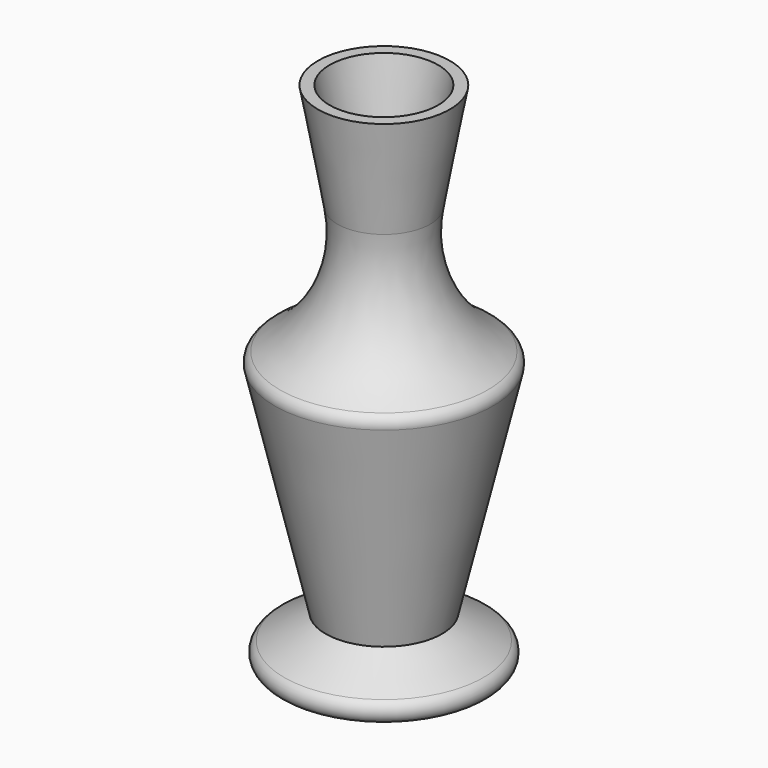
from build123d import *

# Parameters (mm, degrees)
F2_T = -2.54


with BuildPart() as f1:
    # F0 (on Front) → F1 (revolve)
    with BuildSketch(Plane.XZ):
        with BuildLine():
            Line((0, -60.174100101), (0, 52.9934205115))
            Line((0, 52.9934205115), (-14.648579061, 52.9934205115))
            Line((-14.648579061, 52.9934205115), (-10.3401709348, 29.1535649449))
            ThreePointArc((-10.3401709348, 29.1535649449), (-12.3279746399, 13.038394143), (-23.1049332883, 0.8931376273))
            ThreePointArc((-23.1049332883, 0.8931376273), (-24.1326249422, -0.2958024436), (-24.264081516, -1.8618317527))
            Line((-24.264081516, -1.8618317527), (-12.9252169281, -50.1211434603))
            Line((-12.9252169281, -50.1211434603), (-22.1473635946, -55.6544318588))
            ThreePointArc((-22.1473635946, -55.6544318588), (-23.2851239867, -58.5221233208), (-20.8163552246, -60.3723486665))
            Line((-20.8163552246, -60.3723486665), (0, -60.174100101))
        make_face()
    revolve(axis=Axis((0, 0, -3.5903397948), (0, 0, -1)))

    # F2
    f2_openings = [f1.faces().sort_by_distance(p)[0] for p in [
        (0, 0, 52.993421),
    ]]
    offset(amount=F2_T, openings=f2_openings, kind=Kind.INTERSECTION)


solid = f1.part
